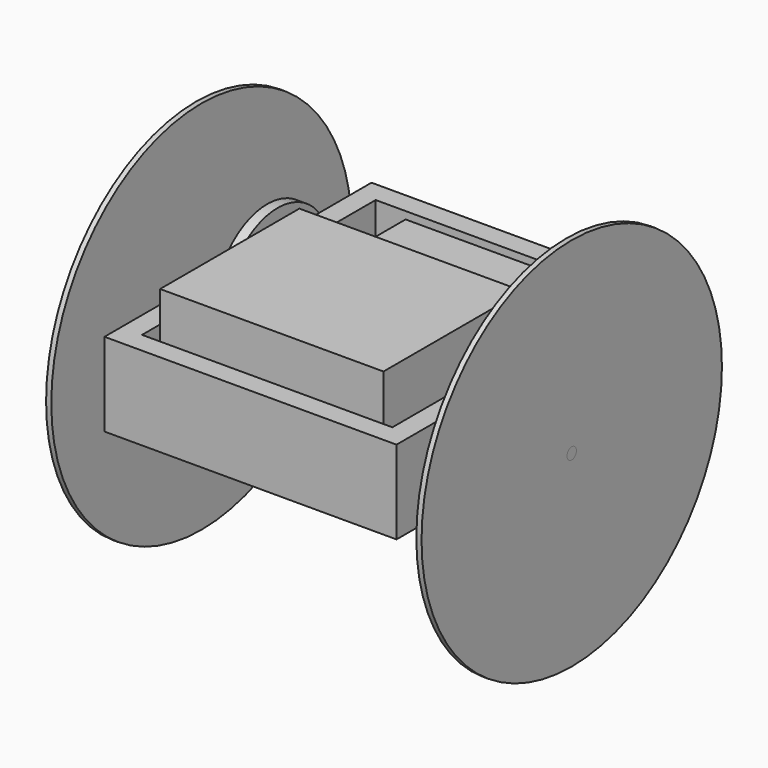
from build123d import *

# Parameters (mm, degrees)
F0_W           = 88.9
F0_H           = 101.6
F0_W_2         = 76.2
F0_H_2         = 88.9
F1_DEPTH       = 25.4
F2_DEPTH       = 3.175
F3_W           = 88.9
F3_H           = 3.175
F4_DEPTH       = 76.2
F5_W           = 47.999904
F5_H           = 25.0000008
F6_DEPTH       = 15.0114
F5_W_2         = 68.000118
F5_H_2         = 52.999894
F7_DEPTH       = 26.0096
F8_R           = 1.7859375
F9_DEPTH       = 6.35
F10_R          = 1.7859375
F11_DEPTH      = 6.35
F12_DEPTH      = 57.15
F12_DEPTH_BACK = 57.15
F15_R          = 57.15
F15_R_2        = 1.7859375
F16_DEPTH      = 1.5875
F17_R          = 57.15
F17_R_2        = 1.7859375
F18_DEPTH      = 1.5875
F20_R          = 1.7859375
F21_DEPTH      = 3.175
F22_R          = 5.0000027
F22_R_2        = 1.7859375
F23_DEPTH      = 3.175
F20_R_2        = 19.99996
F24_DEPTH      = 3.175
F25_DEPTH      = 3.175


# Not quite as in the source:
# - a length typed as a fraction of an inch, garbled in the dataset ("3 / 203.2 mm" for 3/8 in), is restored


with BuildPart() as f1:
    # F0 (on Top) → F1 (new body)
    with BuildSketch(Plane.XY):
        Rectangle(F0_W, F0_H)
        Rectangle(F0_W_2, F0_H_2, mode=Mode.SUBTRACT)
    extrude(amount=F1_DEPTH)

    # F0 (on Top) → F2 (join)
    with BuildSketch(Plane.XY):
        Rectangle(F0_W_2, F0_H_2)
    extrude(amount=F2_DEPTH)

    # F8 (on face) → F9 (cut)
    with BuildSketch(Plane(origin=(-44.45, 0, 0), x_dir=(0, -1, 0), z_dir=(-1, 0, 0))):
        with Locations((0, 6.5484375)):
            Circle(F8_R)
    extrude(amount=-F9_DEPTH, mode=Mode.SUBTRACT)

    # F10 (on face) → F11 (cut)
    with BuildSketch(Plane.YZ.offset(44.45)):
        with Locations((0, 6.5484375)):
            Circle(F10_R)
    extrude(amount=-F11_DEPTH, mode=Mode.SUBTRACT)


with BuildPart() as f4:
    # F3 (on face) → F4 (new body)
    with BuildSketch(Plane.YZ.offset(-38.1)):
        with Locations((0, 10.715625)):
            Rectangle(F3_W, F3_H)
    extrude(amount=F4_DEPTH)


with BuildPart() as f6:
    # F5 (on face) → F6 (new body)
    with BuildSketch(Plane.XY.offset(12.303125)):
        with Locations((0, 25.7093309629)):
            Rectangle(F5_W, F5_H)
    extrude(amount=F6_DEPTH)


with BuildPart() as f7:
    # F5 (on face) → F7 (new body)
    with BuildSketch(Plane.XY.offset(12.303125)):
        with Locations((0, -16.2006690371)):
            Rectangle(F5_W_2, F5_H_2)
    extrude(amount=F7_DEPTH)


with BuildPart() as f12:
    # F8 (on face) → F12 (new body, two sides)
    with BuildSketch(Plane(origin=(-44.45, 0, 0), x_dir=(0, -1, 0), z_dir=(-1, 0, 0))) as f12_sk:
        with Locations((0, 6.5484375)):
            Circle(F8_R)
    extrude(amount=-F12_DEPTH)
    extrude(f12_sk.sketch, amount=F12_DEPTH_BACK)


with BuildPart() as f12_1:
    # F13: moved
    add(f12.part.moved(Location((38.1, 0, 0))))


with BuildPart() as f12_2:
    # F14: moved
    add(f12_1.part.moved(Location((6.35, 0, 0))))


with BuildPart() as f16:
    # F15 (on face) → F16 (new body)
    with BuildSketch(Plane.YZ.offset(57.15)):
        with Locations((0, 6.5484375)):
            Circle(F15_R)
        with Locations((0, 6.5484375)):
            Circle(F15_R_2, mode=Mode.SUBTRACT)
    extrude(amount=-F16_DEPTH)


with BuildPart() as f18:
    # F17 (on face) → F18 (new body)
    with BuildSketch(Plane(origin=(-57.15, 0, 0), x_dir=(0, -1, 0), z_dir=(-1, 0, 0))):
        with Locations((0, 6.5484375)):
            Circle(F17_R)
        with Locations((0, 6.5484375)):
            Circle(F17_R_2, mode=Mode.SUBTRACT)
    extrude(amount=-F18_DEPTH)


with BuildPart() as f21:
    # F20 (on face) → F21 (new body)
    with BuildSketch(Plane(origin=(55.5625, 0, 0), x_dir=(0, -1, 0), z_dir=(-1, 0, 0))):
        with BuildLine():
            ThreePointArc((-5.0000027, 6.5484375), (0, 1.5484348), (5.0000027, 6.5484375))
            ThreePointArc((5.0000027, 6.5484375), (0, 11.5484402), (-5.0000027, 6.5484375))
        make_face()
        with Locations((0, 6.5484375)):
            Circle(F20_R, mode=Mode.SUBTRACT)
    extrude(amount=F21_DEPTH)


with BuildPart() as f23:
    # F22 (on face) → F23 (new body)
    with BuildSketch(Plane.YZ.offset(-55.5625)):
        with Locations((0, 6.5484375)):
            Circle(F22_R)
        with Locations((0, 6.5484375)):
            Circle(F22_R_2, mode=Mode.SUBTRACT)
    extrude(amount=F23_DEPTH)


with BuildPart() as f24:
    # F20 (on face) → F24 (new body)
    with BuildSketch(Plane(origin=(55.5625, 0, 0), x_dir=(0, -1, 0), z_dir=(-1, 0, 0))):
        with Locations((-24.9999627, 6.5484375)):
            Circle(F20_R_2)
    extrude(amount=F24_DEPTH)


with BuildPart() as f25:
    # F22 (on face) → F25 (new body)
    with BuildSketch(Plane.YZ.offset(-55.5625)):
        with BuildLine():
            ThreePointArc((44.9999227, 6.5484375), (24.9999627, 26.5483975), (5.0000027, 6.5484375))
            ThreePointArc((5.0000027, 6.5484375), (24.9999627, -13.4515225), (44.9999227, 6.5484375))
        make_face()
    extrude(amount=F25_DEPTH)


solid = Compound([f1.part, f4.part, f6.part, f7.part, f12_2.part, f16.part, f18.part, f21.part, f23.part, f24.part, f25.part])
